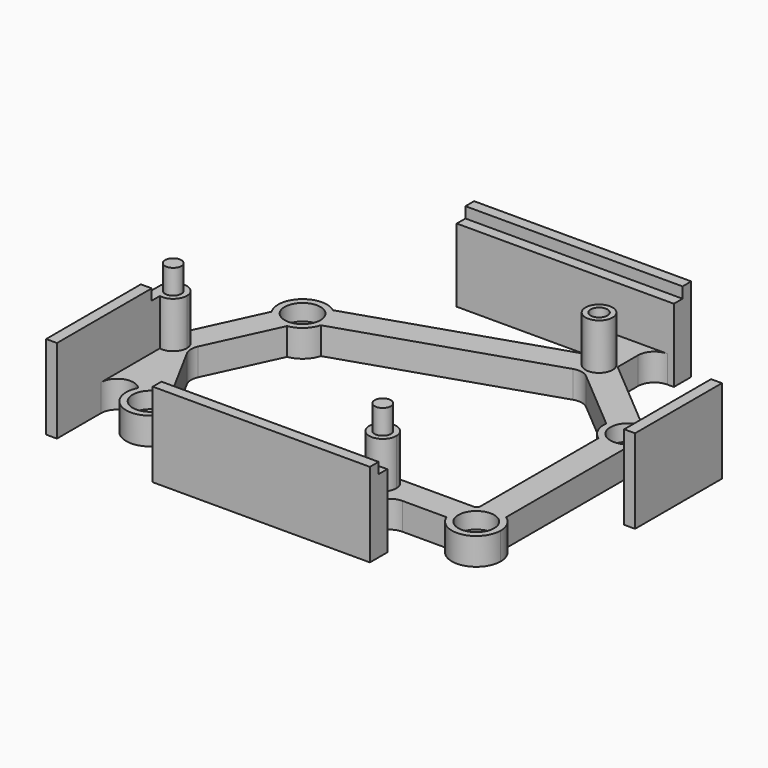
from build123d import *

# Parameters (mm, degrees)
F0_R        = 2.075
F0_R_2      = 1.5
F0_W        = 2
F0_H        = 21.8248448855
F0_R_3      = 1.55
F0_W_2      = 30.8
F0_H_2      = 2
F0_W_3      = 4.2
F0_W_4      = 5
F0_W_5      = 30.55
F1_DEPTH    = 5
F2_W        = 2
F2_H        = 21.8248448855
F2_R        = 2.5
F3_DEPTH    = 8.5
F4_DEPTH    = 11
F5_DEPTH    = 13.5
F6_T1_DEPTH = 5
F7_R        = 3.3
F7_R_2      = 2.075
F8_DEPTH    = 3
F9_DEPTH    = 18
F10_DEPTH   = 15.5


# Not quite as in the source:
# - a fillet or chamfer that OpenCascade refuses, or shapes differently, is made with other operations: its cross-section is extruded or revolved along the edge and cut away or added


with BuildPart() as f1:
    # F0 (on Top) → F1 (new body)
    with BuildSketch(Plane.XY):
        with BuildLine():
            Line((10.8, 24.15), (10.8, 25.9631294877))
            Line((10.8, 25.9631294877), (-27.2199932987, 13.538582024))
            ThreePointArc((-27.2199932987, 13.538582024), (-25.9527768683, 11.967227725), (-25.5, 10))
            ThreePointArc((-25.5, 10), (-25.5419129691, 9.387252071), (-25.666871122, 8.785918402))
            Line((-25.666871122, 8.785918402), (12.7492455063, 21.3399149445))
            Line((12.7492455063, 21.3399149445), (11.6838647694, 22.2426177844))
            ThreePointArc((11.6838647694, 22.2426177844), (11.0317034942, 23.0988906043), (10.8, 24.15))
        make_face()
        with BuildLine():
            ThreePointArc((-27.2199932987, 13.538582024), (-32.9875670099, 13.3651810295), (-33.8429941942, 7.6587619464))
            ThreePointArc((-33.8429941942, 7.6587619464), (-31.8946827733, 5.9183119683), (-29.30778527, 5.5535588649))
            ThreePointArc((-29.30778527, 5.5535588649), (-27.0124329901, 6.6348189705), (-25.666871122, 8.785918402))
            ThreePointArc((-25.666871122, 8.785918402), (-25.5419129691, 9.387252071), (-25.5, 10))
            ThreePointArc((-25.5, 10), (-25.9527768683, 11.967227725), (-27.2199932987, 13.538582024))
        make_face()
        with Locations((-30, 10)):
            Circle(F0_R, mode=Mode.SUBTRACT)
        with BuildLine():
            Line((-33.8429941942, 7.6587619464), (-41.0176044621, -7.7973984593))
            ThreePointArc((-41.0176044621, -7.7973984593), (-38.8274003861, -6.3511984512), (-36.5518888448, -7.6590729035))
            Line((-36.5518888448, -7.6590729035), (-35.9535795759, -8.7633808683))
            Line((-35.9535795759, -8.7633808683), (-29.30778527, 5.5535588649))
            ThreePointArc((-29.30778527, 5.5535588649), (-31.8946827733, 5.9183119683), (-33.8429941942, 7.6587619464))
        make_face()
        with BuildLine():
            ThreePointArc((-41.0176044621, -7.7973984593), (-41.1912098594, -8.3110246551), (-41.25, -8.85))
            ThreePointArc((-41.25, -8.85), (-41.1733528311, -9.4642972049), (-40.9481111552, -10.0409270965))
            ThreePointArc((-40.9481111552, -10.0409270965), (-38.6725996139, -11.3488015488), (-36.4823955379, -9.9026015407))
            ThreePointArc((-36.4823955379, -9.9026015407), (-36.3087901406, -9.3889753449), (-36.25, -8.85))
            ThreePointArc((-36.25, -8.85), (-36.3266471689, -8.2357027951), (-36.5518888448, -7.6590729035))
            ThreePointArc((-36.5518888448, -7.6590729035), (-38.8274003861, -6.3511984512), (-41.0176044621, -7.7973984593))
        make_face()
        with Locations((-38.75, -8.85)):
            Circle(F0_R_2, mode=Mode.SUBTRACT)
        with BuildLine():
            ThreePointArc((-40.9481111552, -10.0409270965), (-41.1733528311, -9.4642972049), (-41.25, -8.85))
            Line((-41.25, -8.85), (-41.25, -13.1751551145))
            Line((-41.25, -13.1751551145), (-39.25, -13.1751551145))
            Line((-39.25, -13.1751551145), (-40.9481111552, -10.0409270965))
        make_face()
        with BuildLine():
            Line((-35.9535795759, -8.7633808683), (-36.5518888448, -7.6590729035))
            ThreePointArc((-36.5518888448, -7.6590729035), (-36.3266471689, -8.2357027951), (-36.25, -8.85))
            ThreePointArc((-36.25, -8.85), (-36.3087901406, -9.3889753449), (-36.4823955379, -9.9026015407))
            Line((-36.4823955379, -9.9026015407), (-35.9535795759, -8.7633808683))
        make_face()
        with BuildLine():
            ThreePointArc((-36.4823955379, -9.9026015407), (-38.6725996139, -11.3488015488), (-40.9481111552, -10.0409270965))
            Line((-40.9481111552, -10.0409270965), (-39.25, -13.1751551145))
            Line((-39.25, -13.1751551145), (-33.9805276223, -22.9010955601))
            ThreePointArc((-33.9805276223, -22.9010955601), (-32.1436687737, -21.0433999206), (-29.5843053118, -20.5192413671))
            Line((-29.5843053118, -20.5192413671), (-35.9535795759, -8.7633808683))
            Line((-35.9535795759, -8.7633808683), (-36.4823955379, -9.9026015407))
        make_face()
        with Locations((-40.25, -24.0875775572)):
            Rectangle(F0_W, F0_H)
        with BuildLine():
            ThreePointArc((-29.5843053118, -20.5192413671), (-32.1436687737, -21.0433999206), (-33.9805276223, -22.9010955601))
            ThreePointArc((-33.9805276223, -22.9010955601), (-31.8528834609, -29.1008319742), (-25.794051831, -26.6))
            ThreePointArc((-25.794051831, -26.6), (-25.5741234337, -25.8133981927), (-25.5, -25))
            ThreePointArc((-25.5, -25), (-25.9063791898, -23.1312387359), (-27.0521194054, -21.6))
            ThreePointArc((-27.0521194054, -21.6), (-28.2335290899, -20.8612102586), (-29.5843053118, -20.5192413671))
        make_face()
        with Locations((-30, -25)):
            Circle(F0_R, mode=Mode.SUBTRACT)
        with BuildLine():
            ThreePointArc((-25.5, -25), (-25.5741234337, -25.8133981927), (-25.794051831, -26.6))
            Line((-25.794051831, -26.6), (10.55, -26.6))
            Line((10.55, -26.6), (10.55, -26.1))
            ThreePointArc((10.55, -26.1), (9.6782917549, -23.309430585), (12.05, -21.6))
            Line((12.05, -21.6), (-27.0521194054, -21.6))
            ThreePointArc((-27.0521194054, -21.6), (-25.9063791898, -23.1312387359), (-25.5, -25))
        make_face()
        with BuildLine():
            Line((10.55, -26.1), (10.55, -26.6))
            Line((10.55, -26.6), (12.05, -26.6))
            ThreePointArc((12.05, -26.6), (11.259430585, -26.4717082451), (10.55, -26.1))
        make_face()
        with BuildLine():
            ThreePointArc((14.5494275812, -24.0465045226), (13.7987511696, -22.3134196501), (12.05, -21.6))
            ThreePointArc((12.05, -21.6), (9.6782917549, -23.309430585), (10.55, -26.1))
            ThreePointArc((10.55, -26.1), (11.259430585, -26.4717082451), (12.05, -26.6))
            ThreePointArc((12.05, -26.6), (13.817766953, -25.867766953), (14.55, -24.1))
            ThreePointArc((14.55, -24.1), (14.5498568912, -24.0732507301), (14.5494275812, -24.0465045226))
        make_face()
        with Locations((12.05, -24.1)):
            Circle(F0_R_2, mode=Mode.SUBTRACT)
        with Locations((12.05, -24.1)):
            Circle(F0_R_2)
        Polygon((12.05, -26.6), (10.55, -26.6), (10.55, -33), (14.7410600647, -33), (14.6040802787, -26.6), align=None)
        with BuildLine():
            ThreePointArc((14.55, -24.1), (13.817766953, -25.867766953), (12.05, -26.6))
            Line((12.05, -26.6), (14.6040802787, -26.6))
            Line((14.6040802787, -26.6), (14.5494275812, -24.0465045226))
            ThreePointArc((14.5494275812, -24.0465045226), (14.5498568912, -24.0732507301), (14.55, -24.1))
        make_face()
        with BuildLine():
            Line((27.0521194054, -21.6), (12.05, -21.6))
            ThreePointArc((12.05, -21.6), (13.7987511696, -22.3134196501), (14.5494275812, -24.0465045226))
            Line((14.5494275812, -24.0465045226), (14.6040802787, -26.6))
            Line((14.6040802787, -26.6), (25.794051831, -26.6))
            ThreePointArc((25.794051831, -26.6), (25.6360205667, -23.9019637959), (27.0521194054, -21.6))
        make_face()
        Polygon((10.55, -35), (-20, -35), (-20, -37), (20, -37), (20, -35), (14.7838662478, -35), align=None)
        with BuildLine():
            ThreePointArc((27.5, -21.2583426132), (27.2707082996, -21.4221561221), (27.0521194054, -21.6))
            ThreePointArc((27.0521194054, -21.6), (25.6360205667, -23.9019637959), (25.794051831, -26.6))
            ThreePointArc((25.794051831, -26.6), (30.8133981927, -29.4258765663), (34.5, -25))
            ThreePointArc((34.5, -25), (33.9686269666, -22.8786796564), (32.5, -21.2583426132))
            ThreePointArc((32.5, -21.2583426132), (30, -20.5), (27.5, -21.2583426132))
        make_face()
        with Locations((30, -25)):
            Circle(F0_R, mode=Mode.SUBTRACT)
        with BuildLine():
            ThreePointArc((32.5, 6.2583426132), (30, 5.5), (27.5, 6.2583426132))
            Line((27.5, 6.2583426132), (27.5, -21.2583426132))
            ThreePointArc((27.5, -21.2583426132), (30, -20.5), (32.5, -21.2583426132))
            Line((32.5, -21.2583426132), (32.5, 6.2583426132))
        make_face()
        with BuildLine():
            ThreePointArc((33.7416573868, 12.5), (31.5492262671, 14.2249139605), (28.761426928, 14.326191945))
            ThreePointArc((28.761426928, 14.326191945), (26.5667120119, 12.9090434151), (25.5291564668, 10.5114275138))
            ThreePointArc((25.5291564668, 10.5114275138), (25.9170662896, 8.1080030877), (27.5, 6.2583426132))
            ThreePointArc((27.5, 6.2583426132), (30, 5.5), (32.5, 6.2583426132))
            ThreePointArc((32.5, 6.2583426132), (33.1819805153, 6.8180194847), (33.7416573868, 7.5))
            ThreePointArc((33.7416573868, 7.5), (34.3062430401, 8.6937569599), (34.5, 10))
            ThreePointArc((34.5, 10), (34.3062430401, 11.3062430401), (33.7416573868, 12.5))
        make_face()
        with Locations((30, 10)):
            Circle(F0_R, mode=Mode.SUBTRACT)
        with BuildLine():
            Line((41.25, 7.5), (41.25, 12.5))
            Line((41.25, 12.5), (33.7416573868, 12.5))
            ThreePointArc((33.7416573868, 12.5), (34.3062430401, 11.3062430401), (34.5, 10))
            ThreePointArc((34.5, 10), (34.3062430401, 8.6937569599), (33.7416573868, 7.5))
            Line((33.7416573868, 7.5), (41.25, 7.5))
        make_face()
        Polygon((43.25, 15), (41.25, 15), (41.25, 12.5), (41.25, 7.5), (41.25, -5), (43.25, -5), align=None)
        with BuildLine():
            ThreePointArc((14.0765610884, 21.773668189), (12.8191677883, 21.6966756464), (11.6838647694, 22.2426177844))
            Line((11.6838647694, 22.2426177844), (12.7492455063, 21.3399149445))
            Line((12.7492455063, 21.3399149445), (14.0765610884, 21.773668189))
        make_face()
        with BuildLine():
            ThreePointArc((14.9161352306, 26.0573822156), (13.7808322117, 26.6033243536), (12.5234389116, 26.526331811))
            ThreePointArc((12.5234389116, 26.526331811), (11.2762160786, 25.6177529218), (10.8, 24.15))
            ThreePointArc((10.8, 24.15), (11.0317034942, 23.0988906043), (11.6838647694, 22.2426177844))
            ThreePointArc((11.6838647694, 22.2426177844), (12.8191677883, 21.6966756464), (14.0765610884, 21.773668189))
            ThreePointArc((14.0765610884, 21.773668189), (15.3237839214, 22.6822470782), (15.8, 24.15))
            ThreePointArc((15.8, 24.15), (15.5682965058, 25.2011093957), (14.9161352306, 26.0573822156))
        make_face()
        with Locations((13.3, 24.15)):
            Circle(F0_R_3, mode=Mode.SUBTRACT)
        with Locations((13.3, 24.15)):
            Circle(F0_R_3)
        with BuildLine():
            Line((28.761426928, 14.326191945), (15.8, 25.3084788332))
            Line((15.8, 25.3084788332), (15.8, 24.15))
            ThreePointArc((15.8, 24.15), (15.3237839214, 22.6822470782), (14.0765610884, 21.773668189))
            Line((14.0765610884, 21.773668189), (12.7492455063, 21.3399149445))
            Line((12.7492455063, 21.3399149445), (25.5291564668, 10.5114275138))
            ThreePointArc((25.5291564668, 10.5114275138), (26.5667120119, 12.9090434151), (28.761426928, 14.326191945))
        make_face()
        with BuildLine():
            Line((12.5234389116, 26.526331811), (10.8, 25.9631294877))
            Line((10.8, 25.9631294877), (10.8, 24.15))
            ThreePointArc((10.8, 24.15), (11.2762160786, 25.6177529218), (12.5234389116, 26.526331811))
        make_face()
        with BuildLine():
            Line((15.8, 24.15), (15.8, 25.3084788332))
            Line((15.8, 25.3084788332), (14.9161352306, 26.0573822156))
            ThreePointArc((14.9161352306, 26.0573822156), (15.5682965058, 25.2011093957), (15.8, 24.15))
        make_face()
        with BuildLine():
            Line((15.8, 33), (10.8, 33))
            Line((10.8, 33), (10.8, 25.9631294877))
            Line((10.8, 25.9631294877), (12.5234389116, 26.526331811))
            ThreePointArc((12.5234389116, 26.526331811), (13.7808322117, 26.6033243536), (14.9161352306, 26.0573822156))
            Line((14.9161352306, 26.0573822156), (15.8, 25.3084788332))
            Line((15.8, 25.3084788332), (15.8, 33))
        make_face()
        Polygon((-20, 37), (-20, 35), (10.8, 35), (15.8, 35), (20, 35), (20, 37), align=None)
        with Locations((-38.75, -8.85)):
            Circle(F0_R_2)
        with Locations((-4.6, 34)):
            Rectangle(F0_W_2, F0_H_2)
        with Locations((17.9, 34)):
            Rectangle(F0_W_3, F0_H_2)
        with Locations((13.3, 34)):
            Rectangle(F0_W_4, F0_H_2)
        Polygon((10.55, -33), (10.55, -35), (14.7838662478, -35), (14.7410600647, -33), align=None)
        Polygon((14.7410600647, -33), (14.7838662478, -35), (20, -35), (20, -33), align=None)
        with Locations((-4.725, -34)):
            Rectangle(F0_W_5, F0_H_2)
    extrude(amount=F1_DEPTH)

    # F2 (on face) → F3 (join)
    with BuildSketch(Plane.XY.offset(5)):
        with Locations((-40.25, -24.0875775572)):
            Rectangle(F2_W, F2_H)
        with BuildLine():
            ThreePointArc((-39.25, -11.2994897428), (-37.1688611699, -10.7864916731), (-36.25, -8.85))
            ThreePointArc((-36.25, -8.85), (-38.2110246551, -6.4087901406), (-41.0176044621, -7.7973984593))
            ThreePointArc((-41.0176044621, -7.7973984593), (-41.1912098594, -8.3110246551), (-41.25, -8.85))
            ThreePointArc((-41.25, -8.85), (-40.6864916731, -10.4311388301), (-39.25, -11.2994897428))
        make_face()
        with Locations((13.3, 24.15)):
            Circle(F2_R)
        Polygon((-20, 33), (10.8, 33), (15.8, 33), (20, 33), (20, 37), (-20, 37), (-20, 35), align=None)
        Polygon((41.25, 15), (41.25, 12.5), (41.25, 7.5), (41.25, -5), (43.25, -5), (43.25, 15), align=None)
        Polygon((14.7410600647, -33), (10.55, -33), (-20, -33), (-20, -37), (20, -37), (20, -33), align=None)
        with BuildLine():
            Line((-39.25, -13.1751551145), (-39.25, -11.2994897428))
            ThreePointArc((-39.25, -11.2994897428), (-40.6864916731, -10.4311388301), (-41.25, -8.85))
            Line((-41.25, -8.85), (-41.25, -13.1751551145))
            Line((-41.25, -13.1751551145), (-39.25, -13.1751551145))
        make_face()
        with BuildLine():
            ThreePointArc((12.05, -21.6), (10.282233047, -25.867766953), (14.55, -24.1))
            ThreePointArc((14.55, -24.1), (13.817766953, -22.332233047), (12.05, -21.6))
        make_face()
    extrude(amount=F3_DEPTH)

    # F0 (on Top) → F4 (join)
    with BuildSketch(Plane.XY):
        with Locations((-40.25, -24.0875775572)):
            Rectangle(F0_W, F0_H)
        Polygon((10.55, -35), (-20, -35), (-20, -37), (20, -37), (20, -35), (14.7838662478, -35), align=None)
        Polygon((-20, 37), (-20, 35), (10.8, 35), (15.8, 35), (20, 35), (20, 37), align=None)
        Polygon((43.25, 15), (41.25, 15), (41.25, 12.5), (41.25, 7.5), (41.25, -5), (43.25, -5), align=None)
        with Locations((-38.75, -8.85)):
            Circle(F0_R_2)
        with Locations((12.05, -24.1)):
            Circle(F0_R_2)
    extrude(amount=F4_DEPTH)

    # F0 (on Top) → F5 (cut, through all)
    with BuildSketch(Plane.XY):
        with Locations((13.3, 24.15)):
            Circle(F0_R_3)
    extrude(amount=F5_DEPTH, mode=Mode.SUBTRACT)

    # F6: fillet of radius 3 on 12 edges, made by hand

    # F6_s2 → F6_t1 (join)
    with BuildSketch(Plane.XY):
        with BuildLine():
            ThreePointArc((-39.25, -24.8631085894), (-37.2968005701, -22.0516661542), (-33.9805276223, -22.9010955601))
            Line((-33.9805276223, -22.9010955601), (-39.25, -13.1751551145))
            Line((-39.25, -13.1751551145), (-39.25, -24.8631085894))
        make_face()
        with BuildLine():
            ThreePointArc((18.8, 33), (16.6786796564, 32.1213203436), (15.8, 30))
            Line((15.8, 30), (15.8, 33))
            Line((15.8, 33), (18.8, 33))
        make_face()
        with BuildLine():
            ThreePointArc((38.2919601084, 12.5), (40.2284517816, 13.2087121525), (41.25, 15))
            Line((41.25, 15), (41.25, 12.5))
            Line((41.25, 12.5), (38.2919601084, 12.5))
        make_face()
        with BuildLine():
            ThreePointArc((41.25, 4.5), (40.3713203436, 6.6213203436), (38.25, 7.5))
            Line((38.25, 7.5), (41.25, 7.5))
            Line((41.25, 7.5), (41.25, 4.5))
        make_face()
        with BuildLine():
            ThreePointArc((17.6775378499, -33), (15.5790364463, -32.1438964199), (14.6782247524, -30.0641945728))
            Line((14.6782247524, -30.0641945728), (14.7410600647, -33))
            Line((14.7410600647, -33), (17.6775378499, -33))
        make_face()
        with BuildLine():
            ThreePointArc((14.6696635157, -29.6641945728), (15.5250801933, -27.5014985964), (17.6689766132, -26.6))
            Line((17.6689766132, -26.6), (14.6040802787, -26.6))
            Line((14.6040802787, -26.6), (14.6696635157, -29.6641945728))
        make_face()
        with BuildLine():
            ThreePointArc((11.1564668077, 20.8194110511), (12.6653387678, 20.9118021022), (14.0277023905, 20.2566715366))
            Line((14.0277023905, 20.2566715366), (12.7492455063, 21.3399149445))
            Line((12.7492455063, 21.3399149445), (11.1564668077, 20.8194110511))
        make_face()
        with BuildLine():
            ThreePointArc((-35.3190004215, -7.3963160613), (-35.5964369255, -8.7523183735), (-35.2356084533, -10.088550426))
            Line((-35.2356084533, -10.088550426), (-35.9535795759, -8.7633808683))
            Line((-35.9535795759, -8.7633808683), (-35.3190004215, -7.3963160613))
        make_face()
        with BuildLine():
            ThreePointArc((7.55, -26.6), (9.6713203436, -27.4786796564), (10.55, -29.6))
            Line((10.55, -29.6), (10.55, -26.6))
            Line((10.55, -26.6), (7.55, -26.6))
        make_face()
        with BuildLine():
            ThreePointArc((10.55, -30), (9.6713203436, -32.1213203436), (7.55, -33))
            Line((7.55, -33), (10.55, -33))
            Line((10.55, -33), (10.55, -30))
        make_face()
        with BuildLine():
            ThreePointArc((10.8, 30), (9.9213203436, 32.1213203436), (7.8, 33))
            Line((7.8, 33), (10.8, 33))
            Line((10.8, 33), (10.8, 30))
        make_face()
        with BuildLine():
            ThreePointArc((8.731873306, 25.2872866997), (10.2285407057, 26.3775813667), (10.8, 28.1388848729))
            Line((10.8, 28.1388848729), (10.8, 25.9631294877))
            Line((10.8, 25.9631294877), (8.731873306, 25.2872866997))
        make_face()
    extrude(amount=F6_T1_DEPTH)

    # F7 (on face) → F8 (cut)
    with BuildSketch(Plane.XY.offset(5)):
        with Locations((-30, 10)):
            Circle(F7_R)
        with Locations((-30, 10)):
            Circle(F7_R_2, mode=Mode.SUBTRACT)
        with Locations((30, 10)):
            Circle(F7_R)
        with Locations((30, 10)):
            Circle(F7_R_2, mode=Mode.SUBTRACT)
        with Locations((-30, -25)):
            Circle(F7_R)
        with Locations((-30, -25)):
            Circle(F7_R_2, mode=Mode.SUBTRACT)
        with Locations((30, -25)):
            Circle(F7_R)
        with Locations((30, -25)):
            Circle(F7_R_2, mode=Mode.SUBTRACT)
    extrude(amount=-F8_DEPTH, mode=Mode.SUBTRACT)

    # F0 (on Top) → F9 (join)
    with BuildSketch(Plane.XY):
        with Locations((12.05, -24.1)):
            Circle(F0_R_2)
        with Locations((-38.75, -8.85)):
            Circle(F0_R_2)
    extrude(amount=F9_DEPTH)

    # F0 (on Top) → F10 (join)
    with BuildSketch(Plane.XY):
        Polygon((10.55, -35), (-20, -35), (-20, -37), (20, -37), (20, -35), (14.7838662478, -35), align=None)
        with Locations((-40.25, -24.0875775572)):
            Rectangle(F0_W, F0_H)
        Polygon((43.25, 15), (41.25, 15), (41.25, 12.5), (41.25, 7.5), (41.25, -5), (43.25, -5), align=None)
        Polygon((-20, 37), (-20, 35), (10.8, 35), (15.8, 35), (20, 35), (20, 37), align=None)
    extrude(amount=F10_DEPTH)


solid = f1.part
